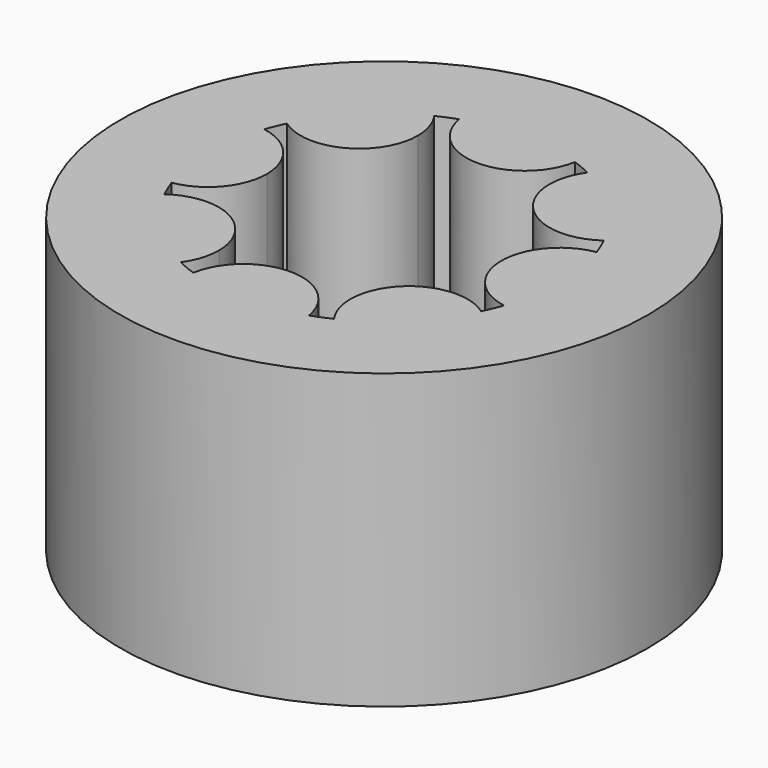
from build123d import *

# Parameters (mm, degrees)
F0_R     = 4.5
F1_DEPTH = 5


with BuildPart() as f1:
    # F0 (on Top) → F1 (new body)
    with BuildSketch(Plane.XY):
        with Locations((0.1191368252, -0.0813986216)):
            Circle(F0_R)
        with BuildLine():
            ThreePointArc((2.8198227273, 1.224853903), (2.8907754227, 1.0666516755), (2.9524701585, 0.9046146756))
            ThreePointArc((2.9524701585, 0.9046146756), (3.7646340496, 0.6823639942), (4.1191368252, -0.0813986216))
            ThreePointArc((4.1191368252, -0.0813986216), (3.7646340496, -0.8451612374), (2.9524701585, -1.0674119188))
            ThreePointArc((2.9524701585, -1.0674119188), (2.8907754227, -1.2294489187), (2.8198227273, -1.3876511462))
            ThreePointArc((2.8198227273, -1.3876511462), (3.129098142, -1.7441154101), (3.2404571688, -2.2027189652))
            ThreePointArc((3.2404571688, -2.2027189652), (2.5445395433, -3.155364707), (1.4253893498, -2.7820845237))
            ThreePointArc((1.4253893498, -2.7820845237), (1.2671871223, -2.8530372191), (1.1051501224, -2.9147319549))
            ThreePointArc((1.1051501224, -2.9147319549), (1.1156340147, -2.9977723613), (1.1191368252, -3.0813986216))
            ThreePointArc((1.1191368252, -3.0813986216), (0.0355105649, -4.0778958111), (-0.866876472, -2.9147319549))
            ThreePointArc((-0.866876472, -2.9147319549), (-1.0289134719, -2.8530372191), (-1.1871156994, -2.7820845237))
            ThreePointArc((-1.1871156994, -2.7820845237), (-2.7092902995, -2.9098257463), (-2.5815490769, -1.3876511462))
            ThreePointArc((-2.5815490769, -1.3876511462), (-2.6525017723, -1.2294489187), (-2.7141965081, -1.0674119188))
            ThreePointArc((-2.7141965081, -1.0674119188), (-3.8808631748, -0.0813986216), (-2.7141965081, 0.9046146756))
            ThreePointArc((-2.7141965081, 0.9046146756), (-2.6525017723, 1.0666516755), (-2.5815490769, 1.224853903))
            ThreePointArc((-2.5815490769, 1.224853903), (-2.7092902995, 2.7470285031), (-1.1871156994, 2.6192872805))
            ThreePointArc((-1.1871156994, 2.6192872805), (-1.0289134719, 2.6902399759), (-0.866876472, 2.7519347117))
            ThreePointArc((-0.866876472, 2.7519347117), (0.0355105649, 3.9150985679), (1.1191368252, 2.9186013784))
            ThreePointArc((1.1191368252, 2.9186013784), (1.1156340147, 2.8349751181), (1.1051501224, 2.7519347117))
            ThreePointArc((1.1051501224, 2.7519347117), (1.2671871223, 2.6902399759), (1.4253893498, 2.6192872805))
            ThreePointArc((1.4253893498, 2.6192872805), (2.5445395433, 2.9925674638), (3.2404571688, 2.039921722))
            ThreePointArc((3.2404571688, 2.039921722), (3.129098142, 1.5813181669), (2.8198227273, 1.224853903))
        make_face(mode=Mode.SUBTRACT)
        with BuildLine():
            ThreePointArc((2.9524701585, -1.0674119188), (3.0771767168, -0.5813986216), (3.1191368252, -0.0813986216))
            ThreePointArc((3.1191368252, -0.0813986216), (3.0771767168, 0.4186013784), (2.9524701585, 0.9046146756))
            ThreePointArc((2.9524701585, 0.9046146756), (2.1191368252, -0.0813986216), (2.9524701585, -1.0674119188))
        make_face()
        with BuildLine():
            ThreePointArc((2.9524701585, 0.9046146756), (3.0771767168, 0.4186013784), (3.1191368252, -0.0813986216))
            ThreePointArc((3.1191368252, -0.0813986216), (3.0771767168, -0.5813986216), (2.9524701585, -1.0674119188))
            ThreePointArc((2.9524701585, -1.0674119188), (3.7646340496, -0.8451612374), (4.1191368252, -0.0813986216))
            ThreePointArc((4.1191368252, -0.0813986216), (3.7646340496, 0.6823639942), (2.9524701585, 0.9046146756))
        make_face()
        with BuildLine():
            ThreePointArc((1.4253893498, 2.6192872805), (1.5333503876, 1.3328149408), (2.8198227273, 1.224853903))
            ThreePointArc((2.8198227273, 1.224853903), (2.2404571688, 2.039921722), (1.4253893498, 2.6192872805))
        make_face()
        with BuildLine():
            ThreePointArc((1.4253893498, 2.6192872805), (2.2404571688, 2.039921722), (2.8198227273, 1.224853903))
            ThreePointArc((2.8198227273, 1.224853903), (3.129098142, 1.5813181669), (3.2404571688, 2.039921722))
            ThreePointArc((3.2404571688, 2.039921722), (2.5445395433, 2.9925674638), (1.4253893498, 2.6192872805))
        make_face()
        with BuildLine():
            ThreePointArc((3.2404571688, -2.2027189652), (3.129098142, -1.7441154101), (2.8198227273, -1.3876511462))
            ThreePointArc((2.8198227273, -1.3876511462), (2.2404571688, -2.2027189652), (1.4253893498, -2.7820845237))
            ThreePointArc((1.4253893498, -2.7820845237), (2.5445395433, -3.155364707), (3.2404571688, -2.2027189652))
        make_face()
        with BuildLine():
            ThreePointArc((1.4253893498, -2.7820845237), (2.2404571688, -2.2027189652), (2.8198227273, -1.3876511462))
            ThreePointArc((2.8198227273, -1.3876511462), (1.5333503876, -1.495612184), (1.4253893498, -2.7820845237))
        make_face()
        with BuildLine():
            ThreePointArc((-0.866876472, 2.7519347117), (0.1191368252, 1.9186013784), (1.1051501224, 2.7519347117))
            ThreePointArc((1.1051501224, 2.7519347117), (0.1191368252, 2.9186013784), (-0.866876472, 2.7519347117))
        make_face()
        with BuildLine():
            ThreePointArc((-0.866876472, 2.7519347117), (0.1191368252, 2.9186013784), (1.1051501224, 2.7519347117))
            ThreePointArc((1.1051501224, 2.7519347117), (1.1156340147, 2.8349751181), (1.1191368252, 2.9186013784))
            ThreePointArc((1.1191368252, 2.9186013784), (0.0355105649, 3.9150985679), (-0.866876472, 2.7519347117))
        make_face()
        with BuildLine():
            ThreePointArc((1.1191368252, -3.0813986216), (1.1156340147, -2.9977723613), (1.1051501224, -2.9147319549))
            ThreePointArc((1.1051501224, -2.9147319549), (0.1191368252, -3.0813986216), (-0.866876472, -2.9147319549))
            ThreePointArc((-0.866876472, -2.9147319549), (0.0355105649, -4.0778958111), (1.1191368252, -3.0813986216))
        make_face()
        with BuildLine():
            ThreePointArc((-0.866876472, -2.9147319549), (0.1191368252, -3.0813986216), (1.1051501224, -2.9147319549))
            ThreePointArc((1.1051501224, -2.9147319549), (0.1191368252, -2.0813986216), (-0.866876472, -2.9147319549))
        make_face()
        with BuildLine():
            ThreePointArc((-1.0021835184, 2.039921722), (-1.0495377765, 2.3440040965), (-1.1871156994, 2.6192872805))
            ThreePointArc((-1.1871156994, 2.6192872805), (-2.0021835184, 2.039921722), (-2.5815490769, 1.224853903))
            ThreePointArc((-2.5815490769, 1.224853903), (-1.5435799633, 1.1512807487), (-1.0021835184, 2.039921722))
        make_face()
        with BuildLine():
            ThreePointArc((-2.5815490769, 1.224853903), (-2.0021835184, 2.039921722), (-1.1871156994, 2.6192872805))
            ThreePointArc((-1.1871156994, 2.6192872805), (-2.7092902995, 2.7470285031), (-2.5815490769, 1.224853903))
        make_face()
        with BuildLine():
            ThreePointArc((-2.5815490769, -1.3876511462), (-2.7092902995, -2.9098257463), (-1.1871156994, -2.7820845237))
            ThreePointArc((-1.1871156994, -2.7820845237), (-2.0021835184, -2.2027189652), (-2.5815490769, -1.3876511462))
        make_face()
        with BuildLine():
            ThreePointArc((-2.5815490769, -1.3876511462), (-2.0021835184, -2.2027189652), (-1.1871156994, -2.7820845237))
            ThreePointArc((-1.1871156994, -2.7820845237), (-1.0495377765, -2.5068013397), (-1.0021835184, -2.2027189652))
            ThreePointArc((-1.0021835184, -2.2027189652), (-1.5435799633, -1.3140779919), (-2.5815490769, -1.3876511462))
        make_face()
        with BuildLine():
            ThreePointArc((-1.8808631748, -0.0813986216), (-2.117100559, 0.5640986028), (-2.7141965081, 0.9046146756))
            ThreePointArc((-2.7141965081, 0.9046146756), (-2.8808631748, -0.0813986216), (-2.7141965081, -1.0674119188))
            ThreePointArc((-2.7141965081, -1.0674119188), (-2.117100559, -0.726895846), (-1.8808631748, -0.0813986216))
        make_face()
        with BuildLine():
            ThreePointArc((-2.7141965081, -1.0674119188), (-2.8808631748, -0.0813986216), (-2.7141965081, 0.9046146756))
            ThreePointArc((-2.7141965081, 0.9046146756), (-3.8808631748, -0.0813986216), (-2.7141965081, -1.0674119188))
        make_face()
    extrude(amount=F1_DEPTH)


solid = f1.part
